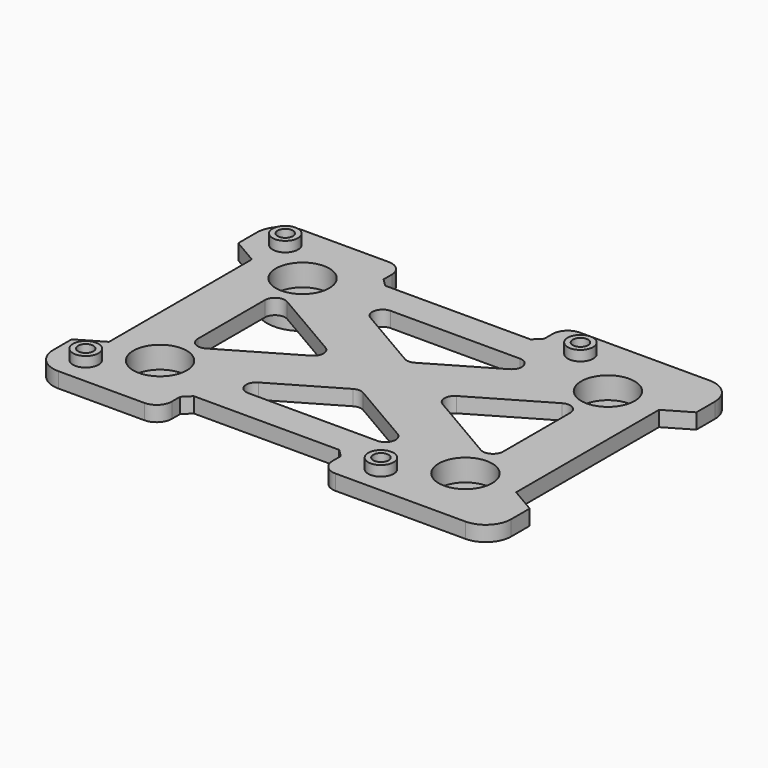
from build123d import *

# Parameters (mm, degrees)
F0_W         = 90
F0_H         = 60
F1_DEPTH     = 3
F2_R         = 2.5
F3_DEPTH     = 2
F4_R         = 1.5
F5_DEPTH     = 5
F6_R         = 7
F7_DEPTH     = 2.5
F8_R         = 5.25
F8_R_2       = 2.1
F9_DEPTH     = 4.3
F10_DEPTH    = 5.5
F11_W        = 31.5768257218
F11_H        = 6.5
F12_DEPTH    = 3
F13_T1_DEPTH = 3
F14_SIZE     = 1.5
F15_R        = 5
F16_R        = 3


# Not quite as in the source:
# - a fillet or chamfer that OpenCascade refuses, or shapes differently, is made with other operations: its cross-section is extruded or revolved along the edge and cut away or added


with BuildPart() as f1:
    # F0 (on Top) → F1 (new body)
    with BuildSketch(Plane.XY):
        Rectangle(F0_W, F0_H)
    extrude(amount=F1_DEPTH)

    # F2 (on face) → F3 (join)
    with BuildSketch(Plane.XY.offset(3)):
        with Locations((-39, 24.5)):
            Circle(F2_R)
        with Locations((19, 24.5)):
            Circle(F2_R)
        with Locations((19, -24.5)):
            Circle(F2_R)
        with Locations((-39, -24.5)):
            Circle(F2_R)
    extrude(amount=F3_DEPTH)

    # F4 (on face) → F5 (cut, through all)
    with BuildSketch(Plane(origin=(0, 0, 0), x_dir=(1, 0, 0), z_dir=(0, 0, -1))):
        with Locations((-39, 24.5)):
            Circle(F4_R)
        with Locations((19, 24.5)):
            Circle(F4_R)
        with Locations((19, -24.5)):
            Circle(F4_R)
        with Locations((-39, -24.5)):
            Circle(F4_R)
    extrude(amount=-F5_DEPTH, mode=Mode.SUBTRACT)

    # F6 (on face) → F7 (join)
    with BuildSketch(Plane(origin=(0, 0, 0), x_dir=(1, 0, 0), z_dir=(0, 0, -1))):
        with Locations((30, -17.5)):
            Circle(F6_R)
        with Locations((30, 17.5)):
            Circle(F6_R)
        with Locations((-30, -17.5)):
            Circle(F6_R)
        with Locations((-30, 17.5)):
            Circle(F6_R)
    extrude(amount=F7_DEPTH)

    # F8 (on face) → F9 (cut)
    with BuildSketch(Plane.XY.offset(3)):
        with Locations((30, -17.5)):
            Circle(F8_R)
        with Locations((30, -17.5)):
            Circle(F8_R_2, mode=Mode.SUBTRACT)
        with Locations((-30, -17.5)):
            Circle(F8_R)
        with Locations((-30, -17.5)):
            Circle(F8_R_2, mode=Mode.SUBTRACT)
        with Locations((-30, 17.5)):
            Circle(F8_R)
        with Locations((-30, 17.5)):
            Circle(F8_R_2, mode=Mode.SUBTRACT)
        with Locations((30, 17.5)):
            Circle(F8_R)
        with Locations((30, 17.5)):
            Circle(F8_R_2, mode=Mode.SUBTRACT)
    extrude(amount=-F9_DEPTH, mode=Mode.SUBTRACT)

    # F8 (on face) → F10 (cut, through all)
    with BuildSketch(Plane.XY.offset(3)):
        with Locations((-30, -17.5)):
            Circle(F8_R_2)
        with Locations((-30, 17.5)):
            Circle(F8_R_2)
        with Locations((30, 17.5)):
            Circle(F8_R_2)
        with Locations((30, -17.5)):
            Circle(F8_R_2)
    extrude(amount=-F10_DEPTH, mode=Mode.SUBTRACT)

    # F11 (on face) → F12 (cut, through all)
    with BuildSketch(Plane.XY.offset(3)):
        Polygon((-40, 17.5448150044), (-45, 20.4614816711), (-45, -20.4614816711), (-40, -17.5448150044), align=None)
        Polygon((-9.9231742782, 0), (-30, 11.7114816711), (-30, -11.7114816711), align=None)
        Polygon((20.0768257218, 17.5), (-20.0768257218, 17.5), (0, 5.7885183289), align=None)
        Polygon((0, -5.7885183289), (-20.0768257218, -17.5), (20.0768257218, -17.5), align=None)
        Polygon((30, 11.7114816711), (9.9231742782, 0), (30, -11.7114816711), align=None)
        Polygon((45, -20.4614816711), (45, 20.4614816711), (40, 17.5448150044), (40, -17.5448150044), align=None)
        with Locations((-4.2884128609, 26.75)):
            Rectangle(F11_W, F11_H)
        with Locations((-4.2884128609, -26.75)):
            Rectangle(F11_W, F11_H)
    extrude(amount=-F12_DEPTH, mode=Mode.SUBTRACT)

    # F13: fillet of radius 2 on 12 edges, made by hand

    # F13_s2 → F13_t1 (join)
    with BuildSketch(Plane.XY):
        with BuildLine():
            ThreePointArc((-26.992257949, -9.9569654746), (-28.9961214529, -9.963691978), (-30, -8.2294076728))
            Line((-30, -8.2294076728), (-30, -11.7114816711))
            Line((-30, -11.7114816711), (-26.992257949, -9.9569654746))
        make_face()
        with BuildLine():
            ThreePointArc((-26.992257949, 9.9569654746), (-28.9961214529, 9.963691978), (-30, 8.2294076728))
            Line((-30, 8.2294076728), (-30, 11.7114816711))
            Line((-30, 11.7114816711), (-26.992257949, 9.9569654746))
        make_face()
        with BuildLine():
            ThreePointArc((-12.8847019384, -1.7275578018), (-11.8924439894, 0), (-12.8847019384, 1.7275578018))
            Line((-12.8847019384, 1.7275578018), (-9.9231742782, 0))
            Line((-9.9231742782, 0), (-12.8847019384, -1.7275578018))
        make_face()
        with BuildLine():
            ThreePointArc((12.8847019384, 1.7275578018), (11.8924439894, 0), (12.8847019384, -1.7275578018))
            Line((12.8847019384, -1.7275578018), (9.9231742782, 0))
            Line((9.9231742782, 0), (12.8847019384, 1.7275578018))
        make_face()
        with BuildLine():
            ThreePointArc((30, -8.2294076728), (28.9961214529, -9.963691978), (26.992257949, -9.9569654746))
            Line((26.992257949, -9.9569654746), (30, -11.7114816711))
            Line((30, -11.7114816711), (30, -8.2294076728))
        make_face()
        with BuildLine():
            ThreePointArc((30, 8.2294076728), (28.9961214529, 9.963691978), (26.992257949, 9.9569654746))
            Line((26.992257949, 9.9569654746), (30, 11.7114816711))
            Line((30, 11.7114816711), (30, 8.2294076728))
        make_face()
        with BuildLine():
            ThreePointArc((12.678984582, 17.5), (14.6096730089, 16.0219599584), (13.686726633, 13.7724421982))
            Line((13.686726633, 13.7724421982), (20.0768257218, 17.5))
            Line((20.0768257218, 17.5), (12.678984582, 17.5))
        make_face()
        with BuildLine():
            ThreePointArc((12.678984582, -17.5), (14.6096730089, -16.0219599584), (13.686726633, -13.7724421982))
            Line((13.686726633, -13.7724421982), (20.0768257218, -17.5))
            Line((20.0768257218, -17.5), (12.678984582, -17.5))
        make_face()
        with BuildLine():
            ThreePointArc((-13.686726633, -13.7724421982), (-14.6096730089, -16.0219599584), (-12.678984582, -17.5))
            Line((-12.678984582, -17.5), (-20.0768257218, -17.5))
            Line((-20.0768257218, -17.5), (-13.686726633, -13.7724421982))
        make_face()
        with BuildLine():
            ThreePointArc((-12.678984582, 17.5), (-14.6096730089, 16.0219599584), (-13.686726633, 13.7724421982))
            Line((-13.686726633, 13.7724421982), (-20.0768257218, 17.5))
            Line((-20.0768257218, 17.5), (-12.678984582, 17.5))
        make_face()
        with BuildLine():
            ThreePointArc((-1.007742051, 6.3763678587), (0, 6.1039256605), (1.007742051, 6.3763678587))
            Line((1.007742051, 6.3763678587), (0, 5.7885183289))
            Line((0, 5.7885183289), (-1.007742051, 6.3763678587))
        make_face()
        with BuildLine():
            ThreePointArc((-1.007742051, -6.3763678587), (0, -6.1039256605), (1.007742051, -6.3763678587))
            Line((1.007742051, -6.3763678587), (0, -5.7885183289))
            Line((0, -5.7885183289), (-1.007742051, -6.3763678587))
        make_face()
    extrude(amount=F13_T1_DEPTH)

    # F14
    f14_edges = [f1.edges().sort_by_distance(p)[0] for p in [
        (11.5, -23.5, 1.5),
        (-20.076826, -23.5, 1.5),
        (11.5, 23.5, 1.5),
        (-20.076826, 23.5, 1.5),
    ]]
    chamfer(f14_edges, length=F14_SIZE)

    # F15
    f15_edges = [f1.edges().sort_by_distance(p)[0] for p in [
        (45, -30, 1.5),
        (45, 30, 1.5),
        (-45, 30, 1.5),
        (-45, -30, 1.5),
    ]]
    fillet(f15_edges, radius=F15_R)

    # F16
    f16_edges = [f1.edges().sort_by_distance(p)[0] for p in [
        (11.5, -30, 1.5),
        (-20.076826, 30, 1.5),
        (11.5, 30, 1.5),
        (-20.076826, -30, 1.5),
    ]]
    fillet(f16_edges, radius=F16_R)


solid = f1.part
